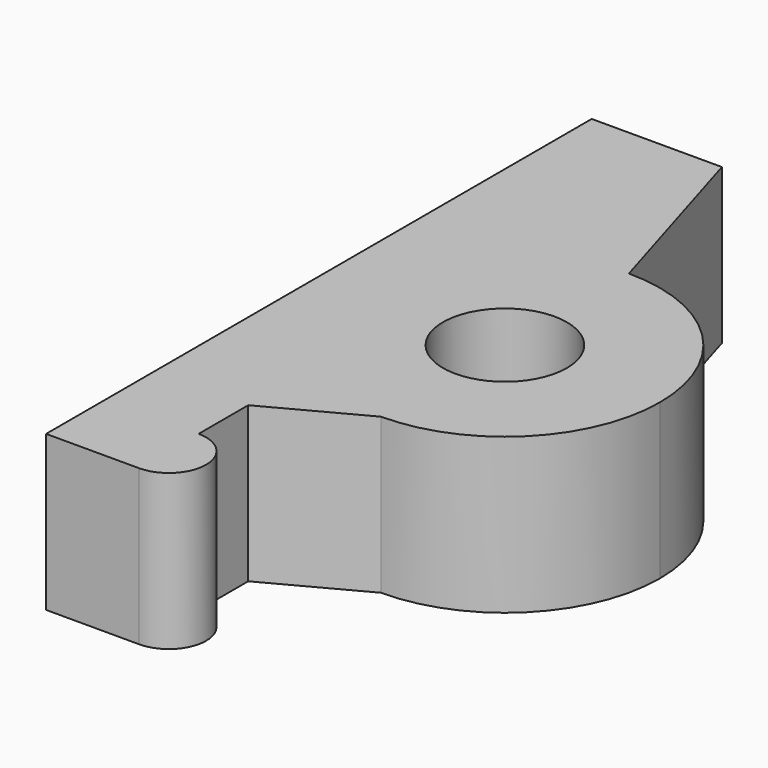
from build123d import *

# Parameters (mm, degrees)
F0_R         = 20
F0_R_2       = 10
F1_DEPTH     = 25
F3_DEPTH     = 5
F2_TEXT_SIZE = 20.4298928093
F4_DEPTH     = 6.1


# Not quite as in the source:
# - Text() gives the source's letters only with a copy of the font that has no kerning and outlines rounded to 1/6400 em; it was checked with that copy


with BuildPart() as f1:
    # F0 (on Top) → F1 (new body)
    with BuildSketch(Plane.XY):
        with BuildLine():
            ThreePointArc((10.3130432405, 13.4427825511), (-7.3646262892, 6.1204520807), (-14.6869567595, -11.5572174489))
            ThreePointArc((-14.6869567595, -11.5572174489), (-7.3646262892, -29.2348869786), (10.3130432405, -36.5572174489))
            ThreePointArc((10.3130432405, -36.5572174489), (27.9907127701, -29.2348869786), (35.3130432405, -11.5572174489))
            ThreePointArc((35.3130432405, -11.5572174489), (27.9907127701, 6.1204520807), (10.3130432405, 13.4427825511))
        make_face()
        with Locations((10.3130432405, -11.5572174489)):
            Circle(F0_R, mode=Mode.SUBTRACT)
        with Locations((10.3130432405, -11.5572174489)):
            Circle(F0_R)
        with Locations((10.3130432405, -11.5572174489)):
            Circle(F0_R_2, mode=Mode.SUBTRACT)
        with BuildLine():
            Line((1.3130432405, 43.4427825511), (-14.6869567595, 43.4427825511))
            Line((-14.6869567595, 43.4427825511), (-14.6869567595, -11.5572174489))
            ThreePointArc((-14.6869567595, -11.5572174489), (-7.3646262892, 6.1204520807), (10.3130432405, 13.4427825511))
            Line((10.3130432405, 13.4427825511), (1.3130432405, 43.4427825511))
        make_face()
        with BuildLine():
            ThreePointArc((10.3130432405, -36.5572174489), (-7.3646262892, -29.2348869786), (-14.6869567595, -11.5572174489))
            Line((-14.6869567595, -11.5572174489), (-14.6869567595, -66.5572174489))
            Line((-14.6869567595, -66.5572174489), (-4.6869567595, -66.5572174489))
            ThreePointArc((-4.6869567595, -66.5572174489), (1.3130432405, -60.5572174489), (-4.6869567595, -54.5572174489))
            Line((-4.6869567595, -54.5572174489), (-4.6869567595, -44.5572174489))
            Line((-4.6869567595, -44.5572174489), (10.3130432405, -36.5572174489))
        make_face()
    extrude(amount=F1_DEPTH)

    # F2 (on face) → F3 (join)
    with BuildSketch(Plane(origin=(-14.6869567595, 0, 0), x_dir=(0, -1, 0), z_dir=(-1, 0, 0))):
        with BuildLine():
            Line((10.1351421359, 1.5162811069), (10.1351421359, 0))
            Line((10.1351421359, 0), (11.4407399732, 0))
            Line((11.4407399732, 0), (16.2896473447, 7.6229037545))
            Line((16.2896473447, 7.6229037545), (11.7695335606, 14.5850281634))
            Line((11.7695335606, 14.5850281634), (13.6465299625, 14.5850281634))
            Line((13.6465299625, 14.5850281634), (17.2664515946, 8.8071991033))
            Line((17.2664515946, 8.8071991033), (20.9182949343, 14.5850281634))
            Line((20.9182949343, 14.5850281634), (22.7218714088, 14.5850281634))
            Line((22.7218714088, 14.5850281634), (18.2049497955, 7.680362828))
            Line((18.2049497955, 7.680362828), (23.0730101915, 0))
            Line((23.0730101915, 0), (31.136048237, 0))
            add(Edge.make_bspline(
                [(31.136048237, 0), (30.2437688993, 0.1802782558), (29.3998926209, 0.5873594183)],
                knots=[0.0691615274, 0.0691615274, 0.0691615274, 1, 1, 1], degree=2))
            Line((29.3998926209, 0.5873594183), (29.3998926209, 2.1642917695))
            add(Edge.make_bspline(
                [(29.3998926209, 2.1642917695), (30.347967334, 1.695042669), (31.4205367065, 1.4508416065)],
                knots=[0, 0, 0, 1, 1, 1], degree=2))
            add(Edge.make_bspline(
                [(31.4205367065, 1.4508416065), (32.493106079, 1.206640544), (33.4507573045, 1.206640544)],
                knots=[0, 0, 0, 1, 1, 1], degree=2))
            add(Edge.make_bspline(
                [(33.4507573045, 1.206640544), (37.2302874742, 1.206640544), (37.2302874742, 4.1689750014)],
                knots=[0, 0, 0, 1, 1, 1], degree=2))
            add(Edge.make_bspline(
                [(37.2302874742, 4.1689750014), (37.2302874742, 6.8248610666), (33.0613124728, 6.8248610666)],
                knots=[0, 0, 0, 1, 1, 1], degree=2))
            Line((33.0613124728, 6.8248610666), (31.6248356346, 6.8248610666))
            Line((31.6248356346, 6.8248610666), (31.6248356346, 8.2485692217))
            Line((31.6248356346, 8.2485692217), (33.0804654973, 8.2485692217))
            add(Edge.make_bspline(
                [(33.0804654973, 8.2485692217), (34.7850846786, 8.2485692217), (35.7826380384, 9.0019215191)],
                knots=[0, 0, 0, 1, 1, 1], degree=2))
            add(Edge.make_bspline(
                [(35.7826380384, 9.0019215191), (36.7801913982, 9.7552738164), (36.7801913982, 11.0927933613)],
                knots=[0, 0, 0, 1, 1, 1], degree=2))
            add(Edge.make_bspline(
                [(36.7801913982, 11.0927933613), (36.7801913982, 12.1589783923), (36.0475882108, 12.7686830058)],
                knots=[0, 0, 0, 1, 1, 1], degree=2))
            add(Edge.make_bspline(
                [(36.0475882108, 12.7686830058), (35.3149850233, 13.3783876193), (34.0572697472, 13.3783876193)],
                knots=[0, 0, 0, 1, 1, 1], degree=2))
            add(Edge.make_bspline(
                [(34.0572697472, 13.3783876193), (33.0996185218, 13.3783876193), (32.2520971873, 13.1182257031)],
                knots=[0, 0, 0, 1, 1, 1], degree=2))
            add(Edge.make_bspline(
                [(32.2520971873, 13.1182257031), (31.4045758528, 12.8580637868), (30.3160456265, 12.1589783923)],
                knots=[0, 0, 0, 1, 1, 1], degree=2))
            Line((30.3160456265, 12.1589783923), (29.4796968896, 13.2762381553))
            add(Edge.make_bspline(
                [(29.4796968896, 13.2762381553), (30.3766968708, 13.9849000621), (31.5482235366, 14.3887096622)],
                knots=[0, 0, 0, 1, 1, 1], degree=2))
            add(Edge.make_bspline(
                [(31.5482235366, 14.3887096622), (32.7197502024, 14.7925192622), (34.0189636982, 14.7925192622)],
                knots=[0, 0, 0, 1, 1, 1], degree=2))
            add(Edge.make_bspline(
                [(34.0189636982, 14.7925192622), (36.1417572479, 14.7925192622), (37.3196682552, 13.8205032684)],
                knots=[0, 0, 0, 1, 1, 1], degree=2))
            add(Edge.make_bspline(
                [(37.3196682552, 13.8205032684), (38.4975792625, 12.8484872746), (38.4975792625, 11.1534446056)],
                knots=[0, 0, 0, 1, 1, 1], degree=2))
            add(Edge.make_bspline(
                [(38.4975792625, 11.1534446056), (38.4975792625, 9.7552738164), (37.713901343, 8.8678503475)],
                knots=[0, 0, 0, 1, 1, 1], degree=2))
            add(Edge.make_bspline(
                [(37.713901343, 8.8678503475), (36.9302234235, 7.9804268786), (35.4937465854, 7.680362828)],
                knots=[0, 0, 0, 1, 1, 1], degree=2))
            Line((35.4937465854, 7.680362828), (35.4937465854, 7.6005585592))
            add(Edge.make_bspline(
                [(35.4937465854, 7.6005585592), (37.2494404987, 7.3834909481), (38.0969618332, 6.4848948816)],
                knots=[0, 0, 0, 1, 1, 1], degree=2))
            add(Edge.make_bspline(
                [(38.0969618332, 6.4848948816), (38.9444831677, 5.586298815), (38.9444831677, 4.1306689524)],
                knots=[0, 0, 0, 1, 1, 1], degree=2))
            add(Edge.make_bspline(
                [(38.9444831677, 4.1306689524), (38.9444831677, 2.0461814517), (37.4984298173, 0.9225373472)],
                knots=[0, 0, 0, 1, 1, 1], degree=2))
            add(Edge.make_bspline(
                [(37.4984298173, 0.9225373472), (36.6641395403, 0.2742588096), (35.4250154101, 0)],
                knots=[0, 0, 0, 0.5769429439, 0.5769429439, 0.5769429439], degree=2))
            Line((35.4250154101, 0), (43.0386898997, 0))
            add(Edge.make_bspline(
                [(43.0386898997, 0), (42.1109749429, 0.1970965524), (41.4694902321, 0.5873594183)],
                knots=[0.5050353738, 0.5050353738, 0.5050353738, 1, 1, 1], degree=2))
            Line((41.4694902321, 0.5873594183), (41.4694902321, 2.183444794))
            add(Edge.make_bspline(
                [(41.4694902321, 2.183444794), (42.1653834559, 1.7365408888), (43.2028389501, 1.4811672287)],
                knots=[0, 0, 0, 1, 1, 1], degree=2))
            add(Edge.make_bspline(
                [(43.2028389501, 1.4811672287), (44.2402944444, 1.2257935686), (45.2490204018, 1.2257935686)],
                knots=[0, 0, 0, 1, 1, 1], degree=2))
            add(Edge.make_bspline(
                [(45.2490204018, 1.2257935686), (47.0047143151, 1.2257935686), (47.9767303089, 2.0541618786)],
                knots=[0, 0, 0, 1, 1, 1], degree=2))
            add(Edge.make_bspline(
                [(47.9767303089, 2.0541618786), (48.9487463027, 2.8825301886), (48.9487463027, 4.4498860275)],
                knots=[0, 0, 0, 1, 1, 1], degree=2))
            add(Edge.make_bspline(
                [(48.9487463027, 4.4498860275), (48.9487463027, 7.5016012659), (45.2107143528, 7.5016012659)],
                knots=[0, 0, 0, 1, 1, 1], degree=2))
            add(Edge.make_bspline(
                [(45.2107143528, 7.5016012659), (44.2626396396, 7.5016012659), (42.6761307761, 7.2111137275)],
                knots=[0, 0, 0, 1, 1, 1], degree=2))
            Line((42.6761307761, 7.2111137275), (41.817436844, 7.7601670968))
            Line((41.817436844, 7.7601670968), (42.3664902133, 14.5850281634))
            Line((42.3664902133, 14.5850281634), (49.6191021606, 14.5850281634))
            Line((49.6191021606, 14.5850281634), (49.6191021606, 13.0591705442))
            Line((49.6191021606, 13.0591705442), (43.7838140269, 13.0591705442))
            Line((43.7838140269, 13.0591705442), (43.4135222197, 8.6795122732))
            add(Edge.make_bspline(
                [(43.4135222197, 8.6795122732), (44.5595115195, 8.9093485673), (45.6991164778, 8.9093485673)],
                knots=[0, 0, 0, 1, 1, 1], degree=2))
            add(Edge.make_bspline(
                [(45.6991164778, 8.9093485673), (48.0038637603, 8.9093485673), (49.3254224514, 7.7665514383)],
                knots=[0, 0, 0, 1, 1, 1], degree=2))
            add(Edge.make_bspline(
                [(49.3254224514, 7.7665514383), (50.6469811425, 6.6237543093), (50.6469811425, 4.6382241019)],
                knots=[0, 0, 0, 1, 1, 1], degree=2))
            add(Edge.make_bspline(
                [(50.6469811425, 4.6382241019), (50.6469811425, 2.3749750391), (49.2057160482, 1.0869341409)],
                knots=[0, 0, 0, 1, 1, 1], degree=2))
            add(Edge.make_bspline(
                [(49.2057160482, 1.0869341409), (48.3339491777, 0.3078468047), (47.0621825996, 0)],
                knots=[0, 0, 0, 0.6048622658, 0.6048622658, 0.6048622658], degree=2))
            Line((47.0621825996, 0), (66.5572174489, 0))
            Line((66.5572174489, 0), (66.5572174489, 25))
            Line((66.5572174489, 25), (-43.4427825511, 25))
            Line((-43.4427825511, 25), (-43.4427825511, 0))
            Line((-43.4427825511, 0), (2.0046832319, 0))
            Line((2.0046832319, 0), (2.0046832319, 14.5850281634))
            Line((2.0046832319, 14.5850281634), (10.1351421359, 14.5850281634))
            Line((10.1351421359, 14.5850281634), (10.1351421359, 13.0783235687))
            Line((10.1351421359, 13.0783235687), (3.6997259009, 13.0783235687))
            Line((3.6997259009, 13.0783235687), (3.6997259009, 8.3794482226))
            Line((3.6997259009, 8.3794482226), (9.7456973042, 8.3794482226))
            Line((9.7456973042, 8.3794482226), (9.7456973042, 6.8823201401))
            Line((9.7456973042, 6.8823201401), (3.6997259009, 6.8823201401))
            Line((3.6997259009, 6.8823201401), (3.6997259009, 1.5162811069))
            Line((3.6997259009, 1.5162811069), (10.1351421359, 1.5162811069))
        make_face()
    extrude(amount=F3_DEPTH)

    # F2 (on face) → F4 (join)
    with BuildSketch(Plane(origin=(-14.6869567595, 0, 0), x_dir=(0, -1, 0), z_dir=(-1, 0, 0))):
        with Locations((0, 0)):
            Text('EX 35', F2_TEXT_SIZE, font='Open Sans', text_align=(TextAlign.LEFT, TextAlign.BOTTOM))
    extrude(amount=F4_DEPTH)


solid = f1.part
